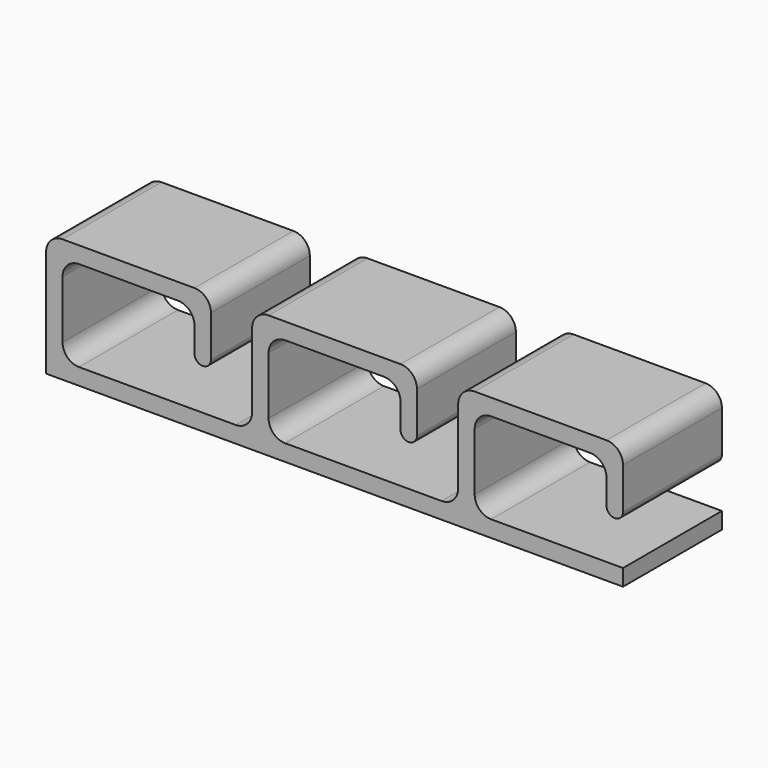
from build123d import *

# Parameters (mm, degrees)
F1_DEPTH = 15
F2_R     = 2
F3_R     = 0.99999
F4_R     = 2


# Not quite as in the source:
# - a fillet or chamfer is up to 0.001 mm smaller than in the source, because OpenCascade refuses the exact size


with BuildPart() as f1:
    # F0 (on Front) → F1 (new body)
    with BuildSketch(Plane.XZ):
        Polygon((-12.5, 15), (-12.5, 0), (57.5, 0), (57.5, 2), (39.5, 2), (39.5, 13), (55.5, 13), (55.5, 7), (57.5, 7), (57.5, 15), (37.5, 15), (37.5, 2), (14.5, 2), (14.5, 13), (30.5, 13), (30.5, 7), (32.5, 7), (32.5, 15), (12.5, 15), (12.5, 2), (-10.5, 2), (-10.5, 13), (5.5, 13), (5.5, 7), (7.5, 7), (7.5, 15), align=None)
    extrude(amount=-F1_DEPTH)

    # F2
    f2_edges = [f1.edges().sort_by_distance(p)[0] for p in [
        (-10.5, 7.5, 2),
        (14.5, 7.5, 2),
        (39.5, 7.5, 2),
        (-10.5, 7.5, 13),
        (14.5, 7.5, 13),
        (39.5, 7.5, 13),
        (37.5, 7.5, 15),
        (12.5, 7.5, 15),
        (-12.5, 7.5, 15),
        (7.5, 7.5, 15),
        (32.5, 7.5, 15),
        (57.5, 7.5, 15),
        (5.5, 7.5, 13),
        (30.5, 7.5, 13),
        (55.5, 7.5, 13),
    ]]
    fillet(f2_edges, radius=F2_R)

    # F3 (radius 1 in the source; OpenCascade refuses exactly that, so slightly less here)
    f3_edges = [f1.edges().sort_by_distance(p)[0] for p in [
        (7.5, 7.5, 7),
        (5.5, 7.5, 7),
        (32.5, 7.5, 7),
        (30.5, 7.5, 7),
        (57.5, 7.5, 7),
        (55.5, 7.5, 7),
    ]]
    fillet(f3_edges, radius=F3_R)

    # F4
    f4_edges = [f1.edges().sort_by_distance(p)[0] for p in [
        (12.5, 7.5, 2),
        (37.5, 7.5, 2),
    ]]
    fillet(f4_edges, radius=F4_R)


solid = f1.part
